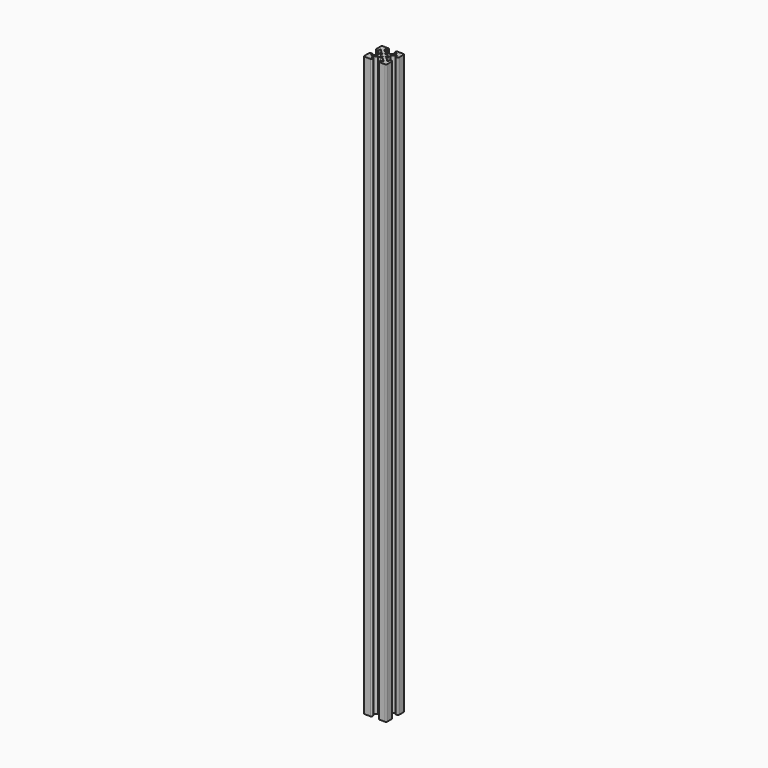
from build123d import *

# Parameters (mm, degrees)
F1_DEPTH = 508
F2_R     = 1
F3_R     = 0.5
F4_R     = 0.1


with BuildPart() as f1:
    # F0 (on Top) → F1 (new body)
    with BuildSketch(Plane.XY):
        with BuildLine():
            Line((-0.025, 4.0583112277), (-2.2905442747, 4.0583112277))
            Line((-2.2905442747, 4.0583112277), (-5.8640526549, 7.6318196079))
            Line((-5.8640526549, 7.6318196079), (-3, 7.6318196079))
            Line((-3, 7.6318196079), (-3, 10))
            Line((-3, 10), (-10, 10))
            Line((-10, 10), (-10, 3))
            Line((-10, 3), (-7.6318196079, 3))
            Line((-7.6318196079, 3), (-7.6318196079, 5.8640526549))
            Line((-7.6318196079, 5.8640526549), (-4, 2.232233047))
            Line((-4, 2.232233047), (-4, 0.025))
            Line((-4, 0.025), (-2.8230957687, 0.025))
            Line((-2.8230957687, 0.025), (-2.8230957687, 0.7926485917))
            Line((-2.8230957687, 0.7926485917), (-1.8740334308, 1.411684829))
            ThreePointArc((-1.8740334308, 1.411684829), (-2.3460869309, 0.0270456781), (-1.906078865, -1.3681077138))
            Line((-1.906078865, -1.3681077138), (-2.8238623803, -0.7794121329))
            Line((-2.8238623803, -0.7794121329), (-2.8238623803, -0.025))
            Line((-2.8238623803, -0.025), (-4, -0.025))
            Line((-4, -0.025), (-4, -2.232233047))
            Line((-4, -2.232233047), (-7.6318196079, -5.8640526549))
            Line((-7.6318196079, -5.8640526549), (-7.6318196079, -3))
            Line((-7.6318196079, -3), (-10, -3))
            Line((-10, -3), (-10, -10))
            Line((-10, -10), (-3, -10))
            Line((-3, -10), (-3, -7.6318196079))
            Line((-3, -7.6318196079), (-5.8640526549, -7.6318196079))
            Line((-5.8640526549, -7.6318196079), (-2.232233047, -4))
            Line((-2.232233047, -4), (-0.05, -4))
            Line((-0.05, -4), (-0.05, -2.9588690959))
            Line((-0.05, -2.9588690959), (-0.7483266194, -2.9588690959))
            Line((-0.7483266194, -2.9588690959), (-1.5537911294, -1.7580069631))
            ThreePointArc((-1.5537911294, -1.7580069631), (-0.0257632285, -2.3461013645), (1.5148107083, -1.7917041816))
            Line((1.5148107083, -1.7917041816), (0.7406048023, -2.9588690959))
            Line((0.7406048023, -2.9588690959), (0.05, -2.9588690959))
            Line((0.05, -2.9588690959), (0.05, -4))
            Line((0.05, -4), (2.232233047, -4))
            Line((2.232233047, -4), (5.8640526549, -7.6318196079))
            Line((5.8640526549, -7.6318196079), (3, -7.6318196079))
            Line((3, -7.6318196079), (3, -10))
            Line((3, -10), (10, -10))
            Line((10, -10), (10, -3))
            Line((10, -3), (7.6318196079, -3))
            Line((7.6318196079, -3), (7.6318196079, -5.8640526549))
            Line((7.6318196079, -5.8640526549), (4, -2.232233047))
            Line((4, -2.232233047), (4, -0.025))
            Line((4, -0.025), (2.8238623803, -0.025))
            Line((2.8238623803, -0.025), (2.8238623803, -0.7921485609))
            Line((2.8238623803, -0.7921485609), (1.8740334308, -1.411684829))
            ThreePointArc((1.8740334308, -1.411684829), (2.3460040432, 0.0334721598), (1.8329957125, 1.4645757318))
            Line((1.8329957125, 1.4645757318), (2.8230957687, 0.8068363719))
            Line((2.8230957687, 0.8068363719), (2.8230957687, 0.025))
            Line((2.8230957687, 0.025), (4, 0.025))
            Line((4, 0.025), (4, 2.232233047))
            Line((4, 2.232233047), (7.6318196079, 5.8640526549))
            Line((7.6318196079, 5.8640526549), (7.6318196079, 3))
            Line((7.6318196079, 3), (10, 3))
            Line((10, 3), (10, 10))
            Line((10, 10), (3, 10))
            Line((3, 10), (3, 7.6318196079))
            Line((3, 7.6318196079), (5.8640526549, 7.6318196079))
            Line((5.8640526549, 7.6318196079), (2.2905442747, 4.0583112277))
            Line((2.2905442747, 4.0583112277), (0.025, 4.0583112277))
            Line((0.025, 4.0583112277), (0.025, 2.9460287187))
            Line((0.025, 2.9460287187), (0.7554459771, 2.9460287187))
            Line((0.7554459771, 2.9460287187), (1.5118729288, 1.7941838266))
            ThreePointArc((1.5118729288, 1.7941838266), (-0.0195250931, 2.3461615731), (-1.5415243666, 1.7687730164))
            Line((-1.5415243666, 1.7687730164), (-0.7608180556, 2.9474266339))
            Line((-0.7608180556, 2.9474266339), (-0.025, 2.9474266339))
            Line((-0.025, 2.9474266339), (-0.025, 4.0583112277))
        make_face()
    extrude(amount=F1_DEPTH)

    # F2
    f2_edges = [f1.edges().sort_by_distance(p)[0] for p in [
        (10, 10, 254),
        (10, -10, 254),
        (-10, -10, 254),
        (-3, -10, 254),
        (3, -10, 254),
        (-3, 10, 254),
        (-10, 3, 254),
        (10, 3, 254),
        (10, -3, 254),
        (-10, -3, 254),
        (-10, 10, 254),
        (3, 10, 254),
    ]]
    fillet(f2_edges, radius=F2_R)

    # F3
    f3_edges = [f1.edges().sort_by_distance(p)[0] for p in [
        (-7.63182, 5.864053, 254),
        (-5.864053, 7.63182, 254),
        (5.864053, 7.63182, 254),
        (7.63182, 5.864053, 254),
        (-7.63182, -5.864053, 254),
        (-5.864053, -7.63182, 254),
        (5.864053, -7.63182, 254),
        (7.63182, -5.864053, 254),
    ]]
    fillet(f3_edges, radius=F3_R)

    # F4
    f4_edges = [f1.edges().sort_by_distance(p)[0] for p in [
        (-1.874033, 1.411685, 254),
        (2.290544, 4.058311, 254),
        (4.656946, 7.63182, 254),
        (-1.541524, 1.768773, 254),
        (1.514811, -1.791704, 254),
        (1.874033, -1.411685, 254),
        (1.832996, 1.464576, 254),
        (1.511873, 1.794184, 254),
        (-1.906079, -1.368108, 254),
        (-1.553791, -1.758007, 254),
    ]]
    fillet(f4_edges, radius=F4_R)


solid = f1.part
